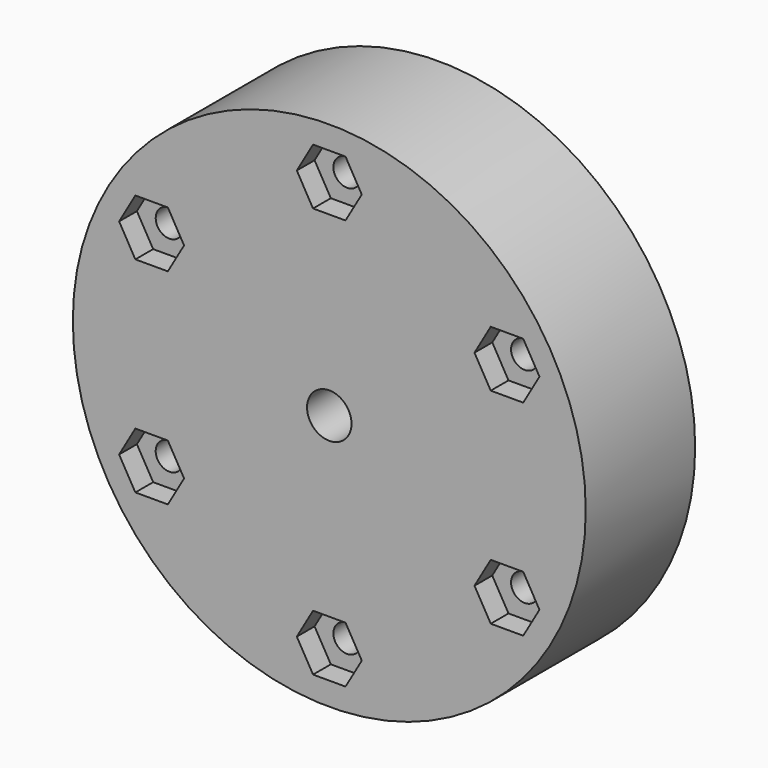
from build123d import *

# Parameters (mm, degrees)
F0_R            = 37.5
F1_DEPTH        = 20
F2_R            = 2
F3_DEPTH        = 20.001
F3_COPIES_COUNT = 6
F5_DEPTH        = 3.25
F5_COPIES_COUNT = 6
F6_R            = 7.5
F7_DEPTH        = 4.15
F8_W            = 7
F8_H            = 7
F9_DEPTH        = 4
F10_W           = 47
F10_H           = 3.18
F11_DEPTH       = 8.15
F12_R           = 3.25
F13_DEPTH       = 11.851


# Not quite as in the source:
# - a pattern or mirror of a feature is missing from the dataset's text; its kind, count and spacing are read off the source's solid


with BuildPart() as f1:
    # F0 (on Front) → F1 (new body)
    with BuildSketch(Plane.XZ):
        Circle(F0_R)
    extrude(amount=F1_DEPTH)

    # F2 (on Front) → F3 (cut, through all)
    with BuildSketch(Plane.XZ):
        with Locations((0, 30)):
            Circle(F2_R)
    f3 = extrude(amount=F3_DEPTH, mode=Mode.SUBTRACT)

    # F3_copies: F3 ×6 about axis
    f3_copies_axis = Axis((0, 0, 0), (0, 1, 0))
    for i in range(1, F3_COPIES_COUNT):
        add(f3.rotate(f3_copies_axis, i * 360 / F3_COPIES_COUNT), mode=Mode.SUBTRACT)

    # F4 (on face) → F5 (cut)
    with BuildSketch(Plane.XZ.offset(20)):
        Polygon((2.3749, 34.1134474629), (-2.3749, 34.1134474629), (-4.7498, 30), (-2.3749, 25.8865525371), (2.3749, 25.8865525371), (4.7498, 30), align=None)
    f5 = extrude(amount=-F5_DEPTH, mode=Mode.SUBTRACT)

    # F5_copies: F5 ×6 about axis
    f5_copies_axis = Axis((0, 0, 0), (0, 1, 0))
    for i in range(1, F5_COPIES_COUNT):
        add(f5.rotate(f5_copies_axis, i * 360 / F5_COPIES_COUNT), mode=Mode.SUBTRACT)

    # F6 (on face) → F7 (cut)
    with BuildSketch(Plane(origin=(0, 0, 0), x_dir=(-1, 0, 0), z_dir=(0, 1, 0))):
        Circle(F6_R)
    extrude(amount=-F7_DEPTH, mode=Mode.SUBTRACT)

    # F8 (on face) → F9 (cut)
    with BuildSketch(Plane(origin=(0, -4.15, 0), x_dir=(-1, 0, 0), z_dir=(0, 1, 0))):
        Rectangle(F8_W, F8_H)
    extrude(amount=-F9_DEPTH, mode=Mode.SUBTRACT)

    # F10 (on face) → F11 (cut, through all)
    with BuildSketch(Plane(origin=(0, 0, 0), x_dir=(-1, 0, 0), z_dir=(0, 1, 0))):
        Rectangle(F10_W, F10_H)
    extrude(amount=-F11_DEPTH, mode=Mode.SUBTRACT)

    # F12 (on face) → F13 (cut, through all)
    with BuildSketch(Plane(origin=(0, -8.15, 0), x_dir=(-1, 0, 0), z_dir=(0, 1, 0))):
        Circle(F12_R)
    extrude(amount=-F13_DEPTH, mode=Mode.SUBTRACT)


solid = f1.part
